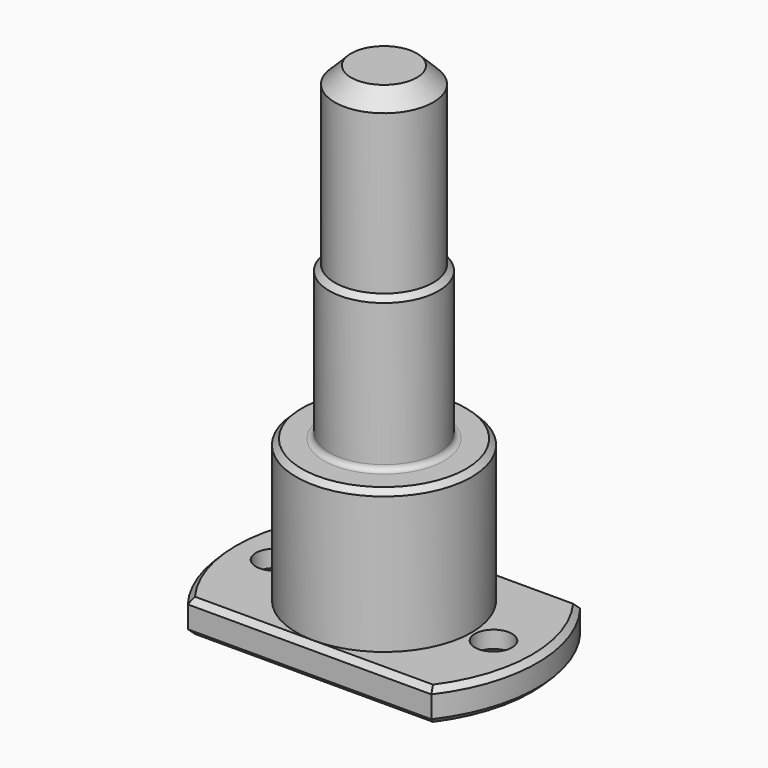
from build123d import *

# Parameters (mm, degrees)
F1_DEPTH        = 3
F2_R            = 8
F3_DEPTH        = 16
F4_R            = 5
F5_DEPTH        = 30
F6_R            = 4.5
F7_DEPTH        = 46
F10_D           = 3.4
F10_CSINK_D     = 6.3
F10_CSINK_ANGLE = 90
F12_SIZE2       = 1.5
F12_SIZE        = 1.5
F13_SIZE2       = 0.49999
F13_SIZE        = 0.49999
F14_SIZE2       = 0.5
F14_SIZE        = 0.5
F15_SIZE2       = 0.49999
F15_SIZE        = 0.49999
F16_SIZE2       = 0.5
F16_SIZE        = 0.5
F17_SIZE2       = 0.49999
F17_SIZE        = 0.49999
F18_SIZE2       = 0.5
F18_SIZE        = 0.5
F19_R           = 0.5
F20_SIZE2       = 0.5
F20_SIZE        = 0.5
F21_SIZE2       = 0.5
F21_SIZE        = 0.5
F22_SIZE2       = 0.5
F22_SIZE        = 0.5
F23_SIZE2       = 0.5
F23_SIZE        = 0.5


# Not quite as in the source:
# - a fillet or chamfer is up to 0.001 mm smaller than in the source, because OpenCascade refuses the exact size
# - a feature of the source that left no trace in its solid (it failed there, or was rolled back) is left out
# - a pattern or mirror of a feature is missing from the dataset's text; its kind, count and spacing are read off the source's solid


with BuildPart() as f1:
    # F0 (on Top) → F1 (new body)
    with BuildSketch(Plane.XY):
        with BuildLine():
            Line((11.1242977306, 8.5), (-11.1242977306, 8.5))
            ThreePointArc((-11.1242977306, 8.5), (-14, 0), (-11.1242977306, -8.5))
            Line((-11.1242977306, -8.5), (11.1242977306, -8.5))
            ThreePointArc((11.1242977306, -8.5), (14, 0), (11.1242977306, 8.5))
        make_face()
    extrude(amount=F1_DEPTH)

    # F2 (on Top) → F3 (join)
    with BuildSketch(Plane.XY):
        Circle(F2_R)
    extrude(amount=F3_DEPTH)

    # F4 (on Top) → F5 (join)
    with BuildSketch(Plane.XY):
        Circle(F4_R)
    extrude(amount=F5_DEPTH)

    # F6 (on Top) → F7 (join)
    with BuildSketch(Plane.XY):
        Circle(F6_R)
    extrude(amount=F7_DEPTH)

    # F10 (through all)
    with Locations(Plane(origin=(0, 0, 0), x_dir=(1, 0, 0), z_dir=(0, 0, -1))):
        with Locations((-10, 0)):
            f10 = CounterSinkHole(F10_D / 2, F10_CSINK_D / 2, counter_sink_angle=F10_CSINK_ANGLE)

    # F10_copies: F10 across plane
    add(f10.mirror(Plane(origin=(0, 0, 0), x_dir=(0, 0, 1), z_dir=(1, 0, 0))), mode=Mode.SUBTRACT)

    # F12
    f12_edges = [f1.edges().sort_by_distance(p)[0] for p in [
        (-4.5, 0, 46),
    ]]
    chamfer(f12_edges, length=F12_SIZE, length2=F12_SIZE2)

    # F13 (size 0.5 and 0.5 in the source; OpenCascade refuses exactly that, so slightly less here)
    f13_edges = [f1.edges().sort_by_distance(p)[0] for p in [
        (-5, 0, 30),
    ]]
    chamfer(f13_edges, length=F13_SIZE, length2=F13_SIZE2)

    # F14
    f14_edges = [f1.edges().sort_by_distance(p)[0] for p in [
        (-8, 0, 16),
    ]]
    chamfer(f14_edges, length=F14_SIZE, length2=F14_SIZE2)

    # F15 (size 0.5 and 0.5 in the source; OpenCascade refuses exactly that, so slightly less here)
    f15_edges = [f1.edges().sort_by_distance(p)[0] for p in [
        (0, -8.5, 3),
    ]]
    chamfer(f15_edges, length=F15_SIZE, length2=F15_SIZE2)

    # F16
    f16_edges = [f1.edges().sort_by_distance(p)[0] for p in [
        (-13.996579, 0.309469, 3),
    ]]
    chamfer(f16_edges, length=F16_SIZE, length2=F16_SIZE2)

    # F17 (size 0.5 and 0.5 in the source; OpenCascade refuses exactly that, so slightly less here)
    f17_edges = [f1.edges().sort_by_distance(p)[0] for p in [
        (0.318105, 8.5, 3),
    ]]
    chamfer(f17_edges, length=F17_SIZE, length2=F17_SIZE2)

    # F18
    f18_edges = [f1.edges().sort_by_distance(p)[0] for p in [
        (14, 0, 3),
    ]]
    chamfer(f18_edges, length=F18_SIZE, length2=F18_SIZE2)

    # F19
    f19_edges = [f1.edges().sort_by_distance(p)[0] for p in [
        (-5, 0, 16),
    ]]
    fillet(f19_edges, radius=F19_R)

    # F20
    f20_edges = [f1.edges().sort_by_distance(p)[0] for p in [
        (0, -8.5, 0),
    ]]
    chamfer(f20_edges, length=F20_SIZE, length2=F20_SIZE2)

    # F21
    f21_edges = [f1.edges().sort_by_distance(p)[0] for p in [
        (-13.996579, 0.309475, 0),
    ]]
    chamfer(f21_edges, length=F21_SIZE, length2=F21_SIZE2)

    # F22
    f22_edges = [f1.edges().sort_by_distance(p)[0] for p in [
        (0.318105, 8.5, 0),
    ]]
    chamfer(f22_edges, length=F22_SIZE, length2=F22_SIZE2)

    # F23
    f23_edges = [f1.edges().sort_by_distance(p)[0] for p in [
        (14, 0, 0),
    ]]
    chamfer(f23_edges, length=F23_SIZE, length2=F23_SIZE2)


solid = f1.part
